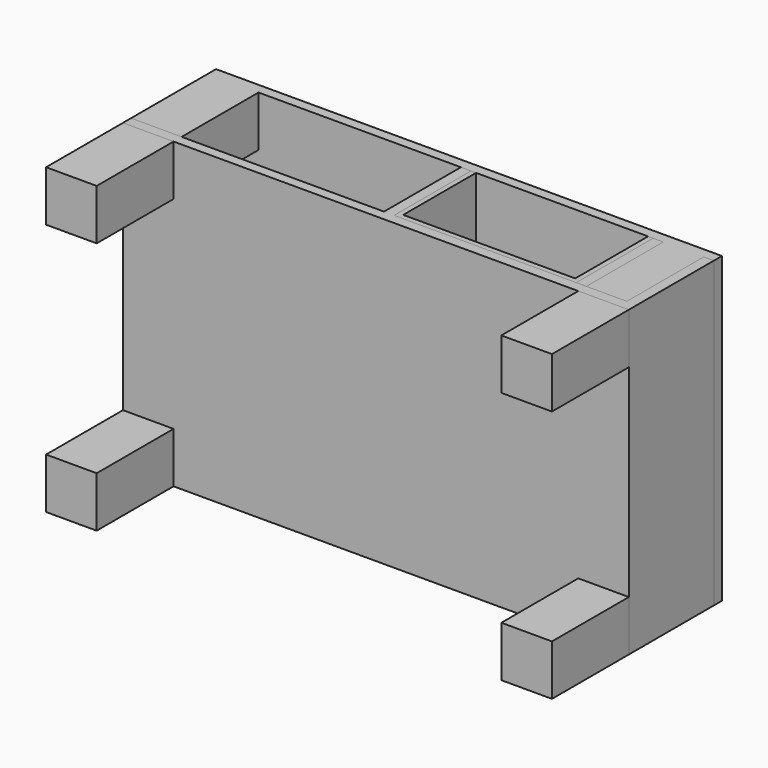
from build123d import *

# Parameters (mm, degrees)
F0_W      = 1000
F0_H      = 600
F1_DEPTH  = 20
F2_W      = 100
F2_H      = 100
F3_DEPTH  = 400
F4_W      = 20
F4_H      = 190
F5_DEPTH  = 300
F6_R      = 40
F7_DEPTH  = 30
F8_R      = 10
F9_DEPTH  = 10
F11_DEPTH = 25.4
F13_DEPTH = 25.4
F14_W     = 190
F14_H     = 600
F14_W_2   = 20
F14_H_2   = 50
F15_DEPTH = 20
F16_W     = 380
F16_H     = 190
F17_DEPTH = 20
F19_DEPTH = 580


# Not quite as in the source:
# - the program builds the solid bodies; features that only make, move or delete a surface that nothing else refers to are left out


with BuildPart() as f1:
    # F0 (on Front) → F1 (new body)
    with BuildSketch(Plane.XZ):
        Rectangle(F0_W, F0_H)
    extrude(amount=F1_DEPTH)

    # F2 (on face) → F3 (join)
    with BuildSketch(Plane.XZ.offset(20)):
        with Locations((450, 250)):
            Rectangle(F2_W, F2_H)
        with Locations((-450, 250)):
            Rectangle(F2_W, F2_H)
        with Locations((450, -250)):
            Rectangle(F2_W, F2_H)
        with Locations((-450, -250)):
            Rectangle(F2_W, F2_H)
    extrude(amount=F3_DEPTH)


with BuildPart() as f5:
    # F4 (on Top) → F5 (new body, symmetric)
    with BuildSketch(Plane.XY):
        Polygon((0, -210), (-500, -210), (-500, -230), (500, -230), (500, -210), (480, -210), (20, -210), align=None)
        with Locations((10, -115)):
            Rectangle(F4_W, F4_H)
        with Locations((490, -115)):
            Rectangle(F4_W, F4_H)
    extrude(amount=F5_DEPTH, both=True)

    # F6 (on face) → F7 (join)
    with BuildSketch(Plane(origin=(480, 0, 0), x_dir=(0, -1, 0), z_dir=(-1, 0, 0))):
        with Locations((115, 0)):
            Circle(F6_R)
    extrude(amount=F7_DEPTH)

    # F8 (on face) → F9 (join)
    with BuildSketch(Plane(origin=(450, 0, 0), x_dir=(0, -1, 0), z_dir=(-1, 0, 0))):
        with Locations((115, 0)):
            Circle(F8_R)
    extrude(amount=F9_DEPTH)


with BuildPart() as f11:
    # F10 (on face) → F11 (new body)
    with BuildSketch(Plane(origin=(440, 0, 0), x_dir=(0, -1, 0), z_dir=(-1, 0, 0))):
        with BuildLine():
            add(Edge.make_bspline(
                [(105.4089282888, 2.8304316686), (108.23936003, 12.4215025071), (89.0572192774, 18.0823691218)],
                knots=[3.1415927352, 3.1415927352, 3.1415927352, 4.7123889804, 4.7123889804, 4.7123889804], degree=2, weights=[1, 0.7071068101, 1]))
            add(Edge.make_bspline(
                [(89.0572192774, 18.0823691218), (42.7474284625, 31.7489119828), (70.6615445509, 5.712223564), (98.5756606394, -20.3244648547), (105.4089282888, 2.8304316686)],
                knots=[4.7123889804, 4.7123889804, 4.7123889804, 7.0685835114, 7.0685835114, 9.4247780424, 9.4247780424, 9.4247780424], degree=2, weights=[1, 0.3826834135, 1, 0.3826834135, 1]))
        make_face()
    extrude(amount=F11_DEPTH)


with BuildPart() as f11b:
    # F10 (on face) → F11, piece 2 (new body)
    with BuildSketch(Plane(origin=(440, 0, 0), x_dir=(0, -1, 0), z_dir=(-1, 0, 0))):
        with BuildLine():
            add(Edge.make_bspline(
                [(123.7749888492, 5.1688648912), (135.7843636375, -7.3121173295), (151.397371578, 19.7292210814), (167.0103795184, 46.7705594923), (139.3879967896, 32.2102033021), (111.7656140609, 17.6498471119), (123.7749888492, 5.1688648912)],
                knots=[0, 0, 0, 2.0943951024, 2.0943951024, 4.1887902048, 4.1887902048, 6.2831853072, 6.2831853072, 6.2831853072], degree=2, weights=[1, 0.5, 1, 0.5, 1, 0.5, 1]))
        make_face()
    extrude(amount=F11_DEPTH)


with BuildPart() as f13:
    # F10 (on face) → F13 (new body)
    with BuildSketch(Plane(origin=(440, 0, 0), x_dir=(0, -1, 0), z_dir=(-1, 0, 0))):
        with BuildLine():
            ThreePointArc((125, 0), (116.4299095929, 9.8972399464), (105.4089282888, 2.8304316686))
            ThreePointArc((105.4089282888, 2.8304316686), (108.4708790022, -7.5743368684), (119.2133449098, -9.0690531298))
            ThreePointArc((119.2133449098, -9.0690531298), (123.4301082169, -5.3789660206), (125, 0))
        make_face()
    extrude(amount=F13_DEPTH)


with BuildPart() as f15:
    # F14 (on face) → F15 (new body)
    with BuildSketch(Plane(origin=(400, 0, 0), x_dir=(0, -1, 0), z_dir=(-1, 0, 0))):
        with Locations((115, 0)):
            Rectangle(F14_W, F14_H)
        with Locations((91.530764699, 25)):
            Rectangle(F14_W_2, F14_H_2, mode=Mode.SUBTRACT)
        with Locations((126.530764699, 25)):
            Rectangle(F14_W_2, F14_H_2, mode=Mode.SUBTRACT)
    extrude(amount=F15_DEPTH)


with BuildPart() as f17:
    # F16 (on face) → F17 (new body)
    with BuildSketch(Plane(origin=(0, 0, -300), x_dir=(1, 0, 0), z_dir=(0, 0, -1))):
        with Locations((210, 115)):
            Rectangle(F16_W, F16_H)
    extrude(amount=-F17_DEPTH)


with BuildPart() as f19:
    # F18 (on face) → F19 (new body)
    with BuildSketch(Plane.XY.offset(-280)):
        Polygon((30, -20), (20, -20), (20, -210), (380, -210), (380, -20), (370, -20), (370, -200), (30, -200), align=None)
    extrude(amount=F19_DEPTH)


solid = Compound([f1.part, f5.part, f11.part, f11b.part, f13.part, f15.part, f17.part, f19.part])
